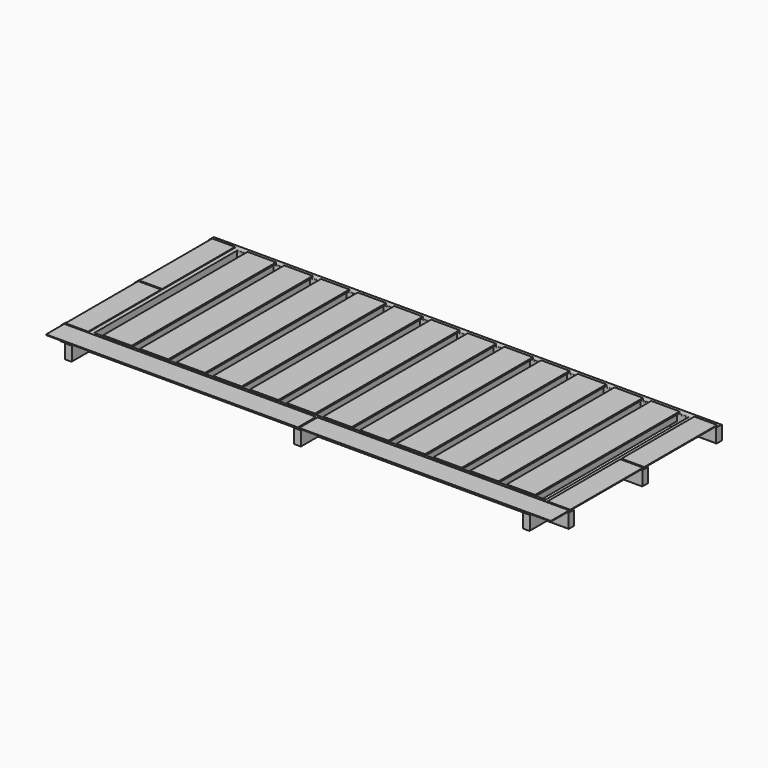
from build123d import *

# Parameters (mm, degrees)
F0_W     = 3170
F0_H     = 1250
F1_DEPTH = 100
F2_R     = 5
F4_W     = 1770
F4_H     = 160
F4_W_2   = 160
F4_H_2   = 640
F5_DEPTH = 5
F6_W     = 50
F6_H     = 1250
F7_DEPTH = 50
F8_W     = 200
F8_H     = 1270
F9_DEPTH = 10


# Not quite as in the source:
# - two fillets or chamfers of one size are made in one step
# - a feature names something its author has since deleted; it is built from what else it names


with BuildPart() as f1:
    # F0 (on Top) → F1 (new body)
    with BuildSketch(Plane.XY):
        Polygon((0, 50), (0, 0), (150, 0), (150, -150), (200, -150), (200, 0), (1760, 0), (1760, -150), (1810, -150), (1810, 0), (3370, 0), (3370, -150), (3420, -150), (3420, 0), (3570, 0), (3570, 50), (3420, 50), (3420, 650), (3420, 700), (3420, 1300), (3570, 1300), (3570, 1350), (0, 1350), (0, 1300), (150, 1300), (150, 700), (150, 650), (150, 50), align=None)
        with Locations((1785, 675)):
            Rectangle(F0_W, F0_H, mode=Mode.SUBTRACT)
        Polygon((0, 650), (150, 650), (150, 700), (0, 700), (0, 675), align=None)
        Polygon((3570, 700), (3420, 700), (3420, 650), (3570, 650), (3570, 675), align=None)
    extrude(amount=-F1_DEPTH)

    # F2
    f2_edges = [f1.edges().sort_by_distance(p)[0] for p in [
        (75, 1300, 0),
        (1785, 1350, 0),
        (1785, 1300, 0),
        (980, 0, 0),
        (1785, 50, 0),
        (75, 50, 0),
        (75, 0, 0),
        (150, -75, 0),
        (3370, 675, 0),
        (3420, 350, 0),
        (3420, 1000, 0),
        (3495, 50, 0),
        (3495, 0, 0),
        (3420, -75, 0),
        (3370, -75, 0),
        (3495, 1300, 0),
        (75, 0, -100),
        (150, -75, -100),
        (200, -75, -100),
        (980, 0, -100),
        (3370, -75, -100),
        (3420, -75, -100),
        (3495, 0, -100),
        (3495, 50, -100),
        (3420, 350, -100),
        (3420, 1000, -100),
        (3495, 1300, -100),
        (1785, 1350, -100),
        (75, 1300, -100),
        (75, 50, -100),
        (1785, 1300, -100),
        (3370, 675, -100),
        (1785, 50, -100),
    ]]
    fillet(f2_edges, radius=F2_R)

    # F4 (on Top) → F5 (join)
    with BuildSketch(Plane.XY):
        with Locations((895, -60)):
            Rectangle(F4_W, F4_H)
        with Locations((2675, -60)):
            Rectangle(F4_W, F4_H)
        with Locations((90, 1000)):
            Rectangle(F4_W_2, F4_H_2)
        with Locations((90, 350)):
            Rectangle(F4_W_2, F4_H_2)
        with Locations((3480, 1000)):
            Rectangle(F4_W_2, F4_H_2)
        with Locations((3480, 350)):
            Rectangle(F4_W_2, F4_H_2)
    extrude(amount=F5_DEPTH)


with BuildPart() as f7:
    # F6 (on Top) → F7 (new body)
    with BuildSketch(Plane.XY):
        with Locations((302, 675)):
            Rectangle(F6_W, F6_H)
    extrude(amount=-F7_DEPTH)


with BuildPart() as f7b:
    # F6 (on Top) → F7, piece 2 (new body)
    with BuildSketch(Plane.XY):
        with Locations((431, 675)):
            Rectangle(F6_W, F6_H)
    extrude(amount=-F7_DEPTH)


with BuildPart() as f7c:
    # F6 (on Top) → F7, piece 3 (new body)
    with BuildSketch(Plane.XY):
        with Locations((560, 675)):
            Rectangle(F6_W, F6_H)
    extrude(amount=-F7_DEPTH)


with BuildPart() as f7d:
    # F6 (on Top) → F7, piece 4 (new body)
    with BuildSketch(Plane.XY):
        with Locations((689, 675)):
            Rectangle(F6_W, F6_H)
    extrude(amount=-F7_DEPTH)


with BuildPart() as f7e:
    # F6 (on Top) → F7, piece 5 (new body)
    with BuildSketch(Plane.XY):
        with Locations((818, 675)):
            Rectangle(F6_W, F6_H)
    extrude(amount=-F7_DEPTH)


with BuildPart() as f7f:
    # F6 (on Top) → F7, piece 6 (new body)
    with BuildSketch(Plane.XY):
        with Locations((947, 675)):
            Rectangle(F6_W, F6_H)
    extrude(amount=-F7_DEPTH)


with BuildPart() as f7g:
    # F6 (on Top) → F7, piece 7 (new body)
    with BuildSketch(Plane.XY):
        with Locations((1076, 675)):
            Rectangle(F6_W, F6_H)
    extrude(amount=-F7_DEPTH)


with BuildPart() as f7h:
    # F6 (on Top) → F7, piece 8 (new body)
    with BuildSketch(Plane.XY):
        with Locations((1205, 675)):
            Rectangle(F6_W, F6_H)
    extrude(amount=-F7_DEPTH)


with BuildPart() as f7i:
    # F6 (on Top) → F7, piece 9 (new body)
    with BuildSketch(Plane.XY):
        with Locations((1334, 675)):
            Rectangle(F6_W, F6_H)
    extrude(amount=-F7_DEPTH)


with BuildPart() as f7j:
    # F6 (on Top) → F7, piece 10 (new body)
    with BuildSketch(Plane.XY):
        with Locations((1463, 675)):
            Rectangle(F6_W, F6_H)
    extrude(amount=-F7_DEPTH)


with BuildPart() as f7k:
    # F6 (on Top) → F7, piece 11 (new body)
    with BuildSketch(Plane.XY):
        with Locations((1592, 675)):
            Rectangle(F6_W, F6_H)
    extrude(amount=-F7_DEPTH)


with BuildPart() as f7l:
    # F6 (on Top) → F7, piece 12 (new body)
    with BuildSketch(Plane.XY):
        with Locations((1721, 675)):
            Rectangle(F6_W, F6_H)
    extrude(amount=-F7_DEPTH)


with BuildPart() as f7m:
    # F6 (on Top) → F7, piece 13 (new body)
    with BuildSketch(Plane.XY):
        with Locations((1850, 675)):
            Rectangle(F6_W, F6_H)
    extrude(amount=-F7_DEPTH)


with BuildPart() as f7n:
    # F6 (on Top) → F7, piece 14 (new body)
    with BuildSketch(Plane.XY):
        with Locations((1979, 675)):
            Rectangle(F6_W, F6_H)
    extrude(amount=-F7_DEPTH)


with BuildPart() as f7o:
    # F6 (on Top) → F7, piece 15 (new body)
    with BuildSketch(Plane.XY):
        with Locations((2108, 675)):
            Rectangle(F6_W, F6_H)
    extrude(amount=-F7_DEPTH)


with BuildPart() as f7p:
    # F6 (on Top) → F7, piece 16 (new body)
    with BuildSketch(Plane.XY):
        with Locations((2237, 675)):
            Rectangle(F6_W, F6_H)
    extrude(amount=-F7_DEPTH)


with BuildPart() as f7q:
    # F6 (on Top) → F7, piece 17 (new body)
    with BuildSketch(Plane.XY):
        with Locations((2366, 675)):
            Rectangle(F6_W, F6_H)
    extrude(amount=-F7_DEPTH)


with BuildPart() as f7r:
    # F6 (on Top) → F7, piece 18 (new body)
    with BuildSketch(Plane.XY):
        with Locations((2495, 675)):
            Rectangle(F6_W, F6_H)
    extrude(amount=-F7_DEPTH)


with BuildPart() as f7s:
    # F6 (on Top) → F7, piece 19 (new body)
    with BuildSketch(Plane.XY):
        with Locations((2624, 675)):
            Rectangle(F6_W, F6_H)
    extrude(amount=-F7_DEPTH)


with BuildPart() as f7t:
    # F6 (on Top) → F7, piece 20 (new body)
    with BuildSketch(Plane.XY):
        with Locations((2753, 675)):
            Rectangle(F6_W, F6_H)
    extrude(amount=-F7_DEPTH)


with BuildPart() as f7u:
    # F6 (on Top) → F7, piece 21 (new body)
    with BuildSketch(Plane.XY):
        with Locations((2882, 675)):
            Rectangle(F6_W, F6_H)
    extrude(amount=-F7_DEPTH)


with BuildPart() as f7v:
    # F6 (on Top) → F7, piece 22 (new body)
    with BuildSketch(Plane.XY):
        with Locations((3011, 675)):
            Rectangle(F6_W, F6_H)
    extrude(amount=-F7_DEPTH)


with BuildPart() as f7w:
    # F6 (on Top) → F7, piece 23 (new body)
    with BuildSketch(Plane.XY):
        with Locations((3140, 675)):
            Rectangle(F6_W, F6_H)
    extrude(amount=-F7_DEPTH)


with BuildPart() as f7x:
    # F6 (on Top) → F7, piece 24 (new body)
    with BuildSketch(Plane.XY):
        with Locations((3269, 675)):
            Rectangle(F6_W, F6_H)
    extrude(amount=-F7_DEPTH)


with BuildPart() as f9:
    # F8 (on Top) → F9 (new body)
    with BuildSketch(Plane.XY):
        with Locations((367, 675)):
            Rectangle(F8_W, F8_H)
    extrude(amount=F9_DEPTH)


with BuildPart() as f9b:
    # F8 (on Top) → F9, piece 2 (new body)
    with BuildSketch(Plane.XY):
        with Locations((625, 675)):
            Rectangle(F8_W, F8_H)
    extrude(amount=F9_DEPTH)


with BuildPart() as f9c:
    # F8 (on Top) → F9, piece 3 (new body)
    with BuildSketch(Plane.XY):
        with Locations((883, 675)):
            Rectangle(F8_W, F8_H)
    extrude(amount=F9_DEPTH)


with BuildPart() as f9d:
    # F8 (on Top) → F9, piece 4 (new body)
    with BuildSketch(Plane.XY):
        with Locations((1141, 675)):
            Rectangle(F8_W, F8_H)
    extrude(amount=F9_DEPTH)


with BuildPart() as f9e:
    # F8 (on Top) → F9, piece 5 (new body)
    with BuildSketch(Plane.XY):
        with Locations((1399, 675)):
            Rectangle(F8_W, F8_H)
    extrude(amount=F9_DEPTH)


with BuildPart() as f9f:
    # F8 (on Top) → F9, piece 6 (new body)
    with BuildSketch(Plane.XY):
        with Locations((1657, 675)):
            Rectangle(F8_W, F8_H)
    extrude(amount=F9_DEPTH)


with BuildPart() as f9g:
    # F8 (on Top) → F9, piece 7 (new body)
    with BuildSketch(Plane.XY):
        with Locations((1915, 675)):
            Rectangle(F8_W, F8_H)
    extrude(amount=F9_DEPTH)


with BuildPart() as f9h:
    # F8 (on Top) → F9, piece 8 (new body)
    with BuildSketch(Plane.XY):
        with Locations((2173, 675)):
            Rectangle(F8_W, F8_H)
    extrude(amount=F9_DEPTH)


with BuildPart() as f9i:
    # F8 (on Top) → F9, piece 9 (new body)
    with BuildSketch(Plane.XY):
        with Locations((2431, 675)):
            Rectangle(F8_W, F8_H)
    extrude(amount=F9_DEPTH)


with BuildPart() as f9j:
    # F8 (on Top) → F9, piece 10 (new body)
    with BuildSketch(Plane.XY):
        with Locations((2689, 675)):
            Rectangle(F8_W, F8_H)
    extrude(amount=F9_DEPTH)


with BuildPart() as f9k:
    # F8 (on Top) → F9, piece 11 (new body)
    with BuildSketch(Plane.XY):
        with Locations((2947, 675)):
            Rectangle(F8_W, F8_H)
    extrude(amount=F9_DEPTH)


with BuildPart() as f9l:
    # F8 (on Top) → F9, piece 12 (new body)
    with BuildSketch(Plane.XY):
        with Locations((3205, 675)):
            Rectangle(F8_W, F8_H)
    extrude(amount=F9_DEPTH)


solid = Compound([f1.part, f7.part, f7b.part, f7c.part, f7d.part, f7e.part, f7f.part, f7g.part, f7h.part, f7i.part, f7j.part, f7k.part, f7l.part, f7m.part, f7n.part, f7o.part, f7p.part, f7q.part, f7r.part, f7s.part, f7t.part, f7u.part, f7v.part, f7w.part, f7x.part, f9.part, f9b.part, f9c.part, f9d.part, f9e.part, f9f.part, f9g.part, f9h.part, f9i.part, f9j.part, f9k.part, f9l.part])
